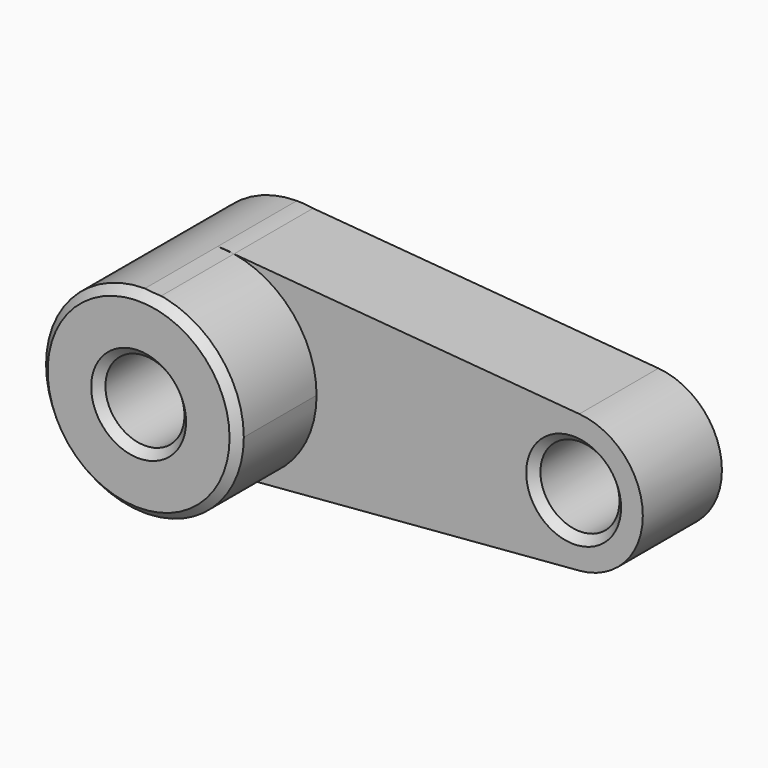
from build123d import *

# Parameters (mm, degrees)
F0_R        = 10
F1_DEPTH    = 25
F2_DEPTH    = 50
F3_T4_ANGLE = 203.6133668192
F3_T6_ANGLE = 179.9906971182


# Not quite as in the source:
# - a fillet or chamfer that OpenCascade refuses, or shapes differently, is made with other operations: its cross-section is extruded or revolved along the edge and cut away or added


with BuildPart() as f1:
    # F0 (on Front) → F1 (new body)
    with BuildSketch(Plane.XZ):
        with BuildLine():
            Line((4.1054428346, 24.6606029758), (0, 25))
            ThreePointArc((0, 25), (-25, 0), (0, -25))
            Line((0, -25), (4.1054428346, -24.6606029758))
            ThreePointArc((4.1054428346, -24.6606029758), (19.0740146648, -16.1611251022), (25, 0))
            ThreePointArc((25, 0), (19.0740146648, 16.1611251022), (4.1054428346, 24.6606029758))
        make_face()
        Circle(F0_R, mode=Mode.SUBTRACT)
        with BuildLine():
            ThreePointArc((4.1054428346, 24.6606029758), (2.0597239626, 24.9150062653), (0, 25))
            Line((0, 25), (4.1054428346, 24.6606029758))
        make_face()
        with BuildLine():
            Line((4.1054428346, -24.6606029758), (0, -25))
            ThreePointArc((0, -25), (2.0597239626, -24.9150062653), (4.1054428346, -24.6606029758))
        make_face()
        with BuildLine():
            Line((91.4418067738, 17.4405043857), (4.1054428346, 24.6606029758))
            ThreePointArc((4.1054428346, 24.6606029758), (19.0740146648, 16.1611251022), (25, 0))
            ThreePointArc((25, 0), (19.0740146648, -16.1611251022), (4.1054428346, -24.6606029758))
            Line((4.1054428346, -24.6606029758), (91.4418067738, -17.4405043857))
            ThreePointArc((91.4418067738, -17.4405043857), (72.5, 0), (91.4418067738, 17.4405043857))
        make_face()
        with BuildLine():
            ThreePointArc((107.5, 0), (102.8740362463, 11.8536572723), (91.4418067738, 17.4405043857))
            ThreePointArc((91.4418067738, 17.4405043857), (72.5, 0), (91.4418067738, -17.4405043857))
            ThreePointArc((91.4418067738, -17.4405043857), (102.8740362463, -11.8536572723), (107.5, 0))
        make_face()
        with Locations((90, 0)):
            Circle(F0_R, mode=Mode.SUBTRACT)
    extrude(amount=F1_DEPTH)

    # F0 (on Front) → F2 (join)
    with BuildSketch(Plane.XZ):
        with BuildLine():
            Line((4.1054428346, 24.6606029758), (0, 25))
            ThreePointArc((0, 25), (-25, 0), (0, -25))
            Line((0, -25), (4.1054428346, -24.6606029758))
            ThreePointArc((4.1054428346, -24.6606029758), (19.0740146648, -16.1611251022), (25, 0))
            ThreePointArc((25, 0), (19.0740146648, 16.1611251022), (4.1054428346, 24.6606029758))
        make_face()
        Circle(F0_R, mode=Mode.SUBTRACT)
    extrude(amount=F2_DEPTH)

    # F3: chamfer of 2 on 4 edges, made by hand

    # F3_s1 → F3_t2 (revolve, cut)
    with BuildSketch(Plane.XY):
        Polygon((12, -50), (10, -48), (10, -50), align=None)
    revolve(axis=Axis((0, -50, 0), (0, -1, 0)), mode=Mode.SUBTRACT)

    # F3_s3 → F3_t4 (revolve, cut)
    with BuildSketch(Plane(origin=(0, 0, 0), x_dir=(0, 1, 0), z_dir=(0.9788435281, 0, -0.2046102329))):
        Polygon((-48, 25), (-50, 23), (-50, 25), align=None)
    revolve(axis=Axis((0, -50, 0), (0, -1, 0)), revolution_arc=F3_T4_ANGLE, mode=Mode.SUBTRACT)

    # F3_s5 → F3_t6 (revolve, cut)
    with BuildSketch(Plane(origin=(0, 0, 0), x_dir=(0, 1, 0), z_dir=(-0.9999999967, 0, 8.1183e-05))):
        Polygon((-48, -25), (-50, -23), (-50, -25), align=None)
    revolve(axis=Axis((0, -50, 0), (0, 1, 0)), revolution_arc=F3_T6_ANGLE, mode=Mode.SUBTRACT)

    # F3_s7 → F3_t8 (revolve, cut)
    with BuildSketch(Plane.XY):
        Polygon((102, -25), (100, -23), (100, -25), align=None)
    revolve(axis=Axis((90, -25, 0), (0, -1, 0)), mode=Mode.SUBTRACT)


solid = f1.part
